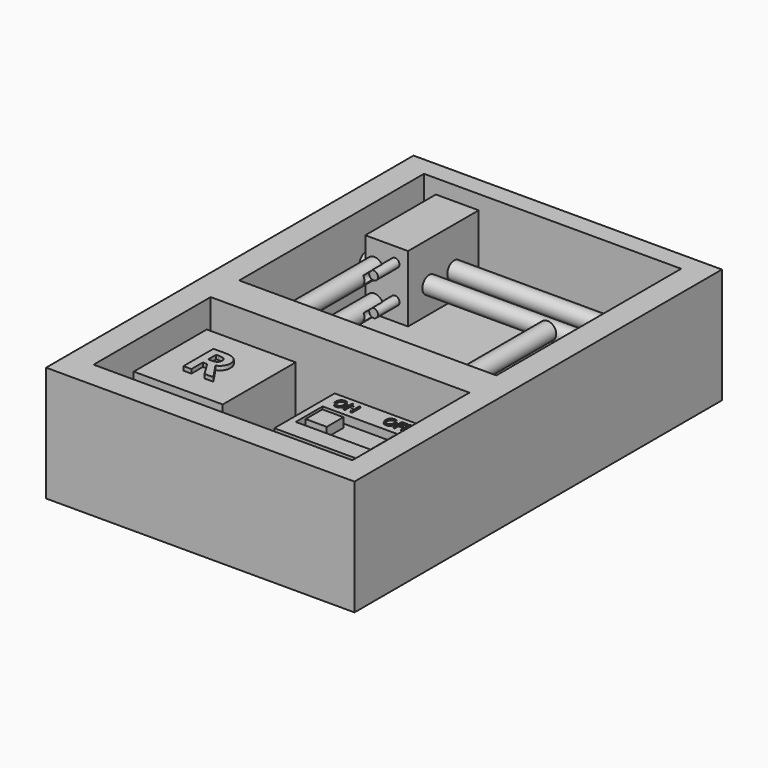
from build123d import *

# Parameters (mm, degrees)
F0_W            = 67.9972469807
F0_H            = 101.2567877769
F1_DEPTH        = 25.4
F2_W            = 57.0491608232
F2_H            = 32.2670452297
F3_DEPTH        = 19.8095608503
F4_W            = 19.6126401424
F4_H            = 20.1155394316
F5_DEPTH        = 17.4587108195
F6_TEXT_SIZE    = 11.5746632218
F7_DEPTH        = 0.8934950456
F8_W            = 20.079113543
F8_H            = 16.6246443987
F9_DEPTH        = 14.8580167443
F10_W           = 16.474539414
F10_H           = 7.4091814458
F11_DEPTH       = 1.836954616
F12_W           = 4.6481993049
F12_H           = 4.6066977084
F13_DEPTH       = 2.0742774941
F14_TEXT_SIZE   = 3.3086709057
F14_TEXT_SIZE_2 = 3.2569928509
F15_DEPTH       = 0.2203329932
F16_W           = 56.6920340061
F16_H           = 50.9403496981
F17_DEPTH       = 17.3227358609
F18_R           = 1.905
F19_DEPTH       = 25.9628873318
F21_START       = 20.7996312529
F20_R           = 0.9525
F21_DEPTH       = 26.1481683701
F22_R           = 1.905
F23_DEPTH       = 58.2528188825
F25_START       = 29.1665140539
F24_W           = 9.4348490238
F24_H           = 14.6446665749
F25_DEPTH       = 19.4627735764
F26_R           = 0.9753499592
F26_R_2         = 0.9671818138
F27_DEPTH       = 25.4


# Not quite as in the source:
# - Text() gives the source's letters only with a copy of the font that has no kerning and outlines rounded to 1/6400 em; it was checked with that copy


with BuildPart() as f1:
    # F0 (on Top) → F1 (new body)
    with BuildSketch(Plane.XY):
        Rectangle(F0_W, F0_H)
    extrude(amount=F1_DEPTH)

    # F2 (on face) → F3 (cut)
    with BuildSketch(Plane.XY.offset(25.4)):
        with Locations((0.2175765112, -28.5167414695)):
            Rectangle(F2_W, F2_H)
    extrude(amount=-F3_DEPTH, mode=Mode.SUBTRACT)

    # F16 (on face) → F17 (cut)
    with BuildSketch(Plane.XY.offset(25.4)):
        with Locations((0, 20.9899693727)):
            Rectangle(F16_W, F16_H)
    extrude(amount=-F17_DEPTH, mode=Mode.SUBTRACT)

    # F18 (on face) → F19 (join)
    with BuildSketch(Plane(origin=(0, -4.4802054763, 0), x_dir=(-1, 0, 0), z_dir=(0, 1, 0))):
        with Locations((-18.8885309738, 20.444400919)):
            Circle(F18_R)
        with Locations((-18.8885309738, 13.3730137962)):
            Circle(F18_R)
        with Locations((19.2825247159, 13.3730137962)):
            Circle(F18_R)
        with Locations((19.2825247159, 20.444400919)):
            Circle(F18_R)
    extrude(amount=F19_DEPTH)

    # F20 (on face) → F21 (cut)
    with BuildSketch(Plane(origin=(0, -4.4802054763, 0), x_dir=(-1, 0, 0), z_dir=(0, 1, 0)).offset(F21_START)):
        with Locations((-16.994740991, 20.5086497498)):
            Circle(F20_R)
        with Locations((-16.994740991, 13.2271844851)):
            Circle(F20_R)
        with Locations((17.3121424871, 13.2271844851)):
            Circle(F20_R)
        with Locations((17.3121424871, 20.5086497498)):
            Circle(F20_R)
    extrude(amount=F21_DEPTH, mode=Mode.SUBTRACT)

    # F22 (on face) → F23 (join)
    with BuildSketch(Plane.YZ.offset(-28.3460170031)):
        with Locations((30.5222657385, 14.8940153793)):
            Circle(F22_R)
        with Locations((37.4011246481, 14.8940153793)):
            Circle(F22_R)
    extrude(amount=F23_DEPTH)


with BuildPart() as f5:
    # F4 (on face) → F5 (new body)
    with BuildSketch(Plane.XY.offset(5.5904391497)):
        with Locations((-14.3059305847, -28.768055141)):
            Rectangle(F4_W, F4_H)
    extrude(amount=F5_DEPTH)


with BuildPart() as f7:
    # F6 (on face) → F7 (new body)
    with BuildSketch(Plane.XY.offset(23.0491499692)):
        with Locations((-18.6795499176, -33.2238376141)):
            Text('R', F6_TEXT_SIZE, font='Open Sans', font_style=FontStyle.BOLD, text_align=(TextAlign.LEFT, TextAlign.BOTTOM))
    extrude(amount=F7_DEPTH)


with BuildPart() as f9:
    # F8 (on face) → F9 (new body)
    with BuildSketch(Plane.XY.offset(5.5904391497)):
        with Locations((14.8919075727, -27.9701165855)):
            Rectangle(F8_W, F8_H)
    extrude(amount=F9_DEPTH)

    # F10 (on face) → F11 (cut)
    with BuildSketch(Plane.XY.offset(20.448455894)):
        with Locations((14.5025318488, -28.4504611045)):
            Rectangle(F10_W, F10_H)
    extrude(amount=-F11_DEPTH, mode=Mode.SUBTRACT)


with BuildPart() as f13:
    # F12 (on face) → F13 (new body)
    with BuildSketch(Plane.XY.offset(18.611501278)):
        with Locations((9.5375701785, -28.3053237945)):
            Rectangle(F12_W, F12_H)
    extrude(amount=F13_DEPTH)


with BuildPart() as f15:
    # F14 (on face) → F15 (new body)
    with BuildSketch(Plane.XY.offset(20.448455894)):
        with Locations((6.9536343217, -23.4318189323)):
            Text('ON', F14_TEXT_SIZE, font='Open Sans', text_align=(TextAlign.LEFT, TextAlign.BOTTOM))
        with Locations((17.9518926889, -23.4044082463)):
            Text('OFF', F14_TEXT_SIZE_2, font='Open Sans', text_align=(TextAlign.LEFT, TextAlign.BOTTOM))
    extrude(amount=F15_DEPTH)


with BuildPart() as f25:
    # F24 (on face) → F25 (new body)
    with BuildSketch(Plane(origin=(0, -4.4802054763, 0), x_dir=(-1, 0, 0), z_dir=(0, 1, 0)).offset(F25_START)):
        with Locations((19.1614031792, 16.4485615678)):
            Rectangle(F24_W, F24_H)
    extrude(amount=F25_DEPTH)

    # F26 (on face) → F27 (join)
    with BuildSketch(Plane(origin=(0, 44.149082154, 0), x_dir=(-1, 0, 0), z_dir=(0, 1, 0))):
        with Locations((17.306547612, 13.220560737)):
            Circle(F26_R)
        with Locations((17.306547612, 20.5372590572)):
            Circle(F26_R_2)
    extrude(amount=-F27_DEPTH)


solid = Compound([f1.part, f5.part, f7.part, f9.part, f13.part, f15.part, f25.part])
